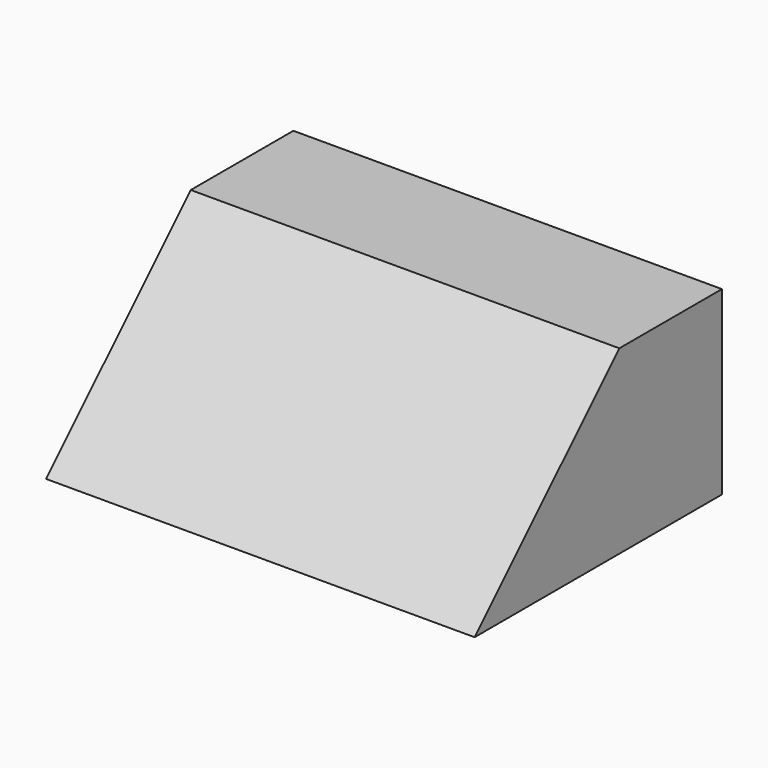
from build123d import *

# Parameters (mm, degrees)
F0_W     = 118.4879094362
F0_H     = 85.4637138546
F1_DEPTH = 50
F2_SIZE  = 49.99999


# Not quite as in the source:
# - a fillet or chamfer is up to 0.001 mm smaller than in the source, because OpenCascade refuses the exact size


with BuildPart() as f1:
    # F0 (on Top) → F1 (new body)
    with BuildSketch(Plane.XY):
        with Locations((0.7258094847, -1.0887105018)):
            Rectangle(F0_W, F0_H)
    extrude(amount=F1_DEPTH)

    # F2 (size 50 in the source; OpenCascade refuses exactly that, so slightly less here)
    f2_edges = [f1.edges().sort_by_distance(p)[0] for p in [
        (0.725809, -43.820567, 50),
    ]]
    chamfer(f2_edges, length=F2_SIZE)


solid = f1.part
